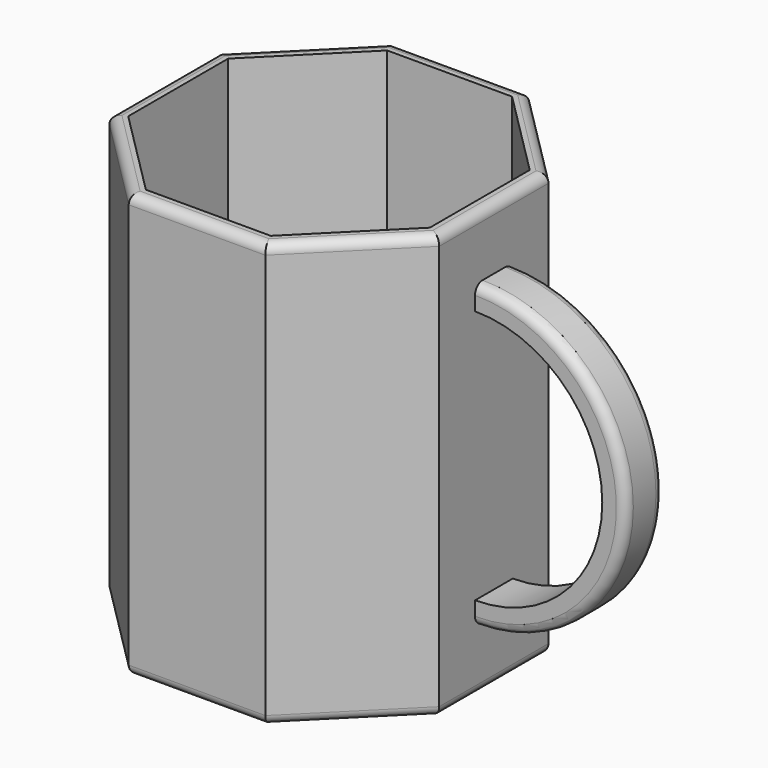
from build123d import *

# Parameters (mm, degrees)
F1_DEPTH      = 90
F2_DEPTH      = 5
F4_DEPTH      = 5
F4_DEPTH_BACK = 5
F5_R          = 2
F5_2_R        = 2


# Not quite as in the source:
# - a feature names something its author has since deleted; it is built from what else it names


with BuildPart() as f1:
    # F0 (on Top) → F1 (new body)
    with BuildSketch(Plane.XY):
        Polygon((14.4974746831, 35), (-14.4974746831, 35), (-35, 14.4974746831), (-35, -14.4974746831), (-14.4974746831, -35), (14.4974746831, -35), (35, -14.4974746831), (35, 14.4974746831), align=None)
        Polygon((-32, 13.2548339959), (-13.2548339959, 32), (13.2548339959, 32), (32, 13.2548339959), (32, -13.2548339959), (13.2548339959, -32), (-13.2548339959, -32), (-32, -13.2548339959), align=None, mode=Mode.SUBTRACT)
    extrude(amount=F1_DEPTH)

    # F5
    f5_edges = [f1.edges().sort_by_distance(p)[0] for p in [
        (24.748737, 24.748737, 90),
        (0, 35, 90),
        (-24.748737, 24.748737, 90),
        (-35, 0, 90),
        (-24.748737, -24.748737, 90),
        (0, -35, 90),
        (24.748737, -24.748737, 90),
        (35, 0, 90),
        (35, 0, 0),
        (24.748737, 24.748737, 0),
        (0, 35, 0),
        (-24.748737, 24.748737, 0),
        (-35, 0, 0),
        (-24.748737, -24.748737, 0),
        (0, -35, 0),
        (24.748737, -24.748737, 0),
    ]]
    fillet(f5_edges, radius=F5_R)


with BuildPart() as f2:
    # F0 (on Top) → F2 (new body)
    with BuildSketch(Plane.XY):
        Polygon((13.2548339959, 32), (-13.2548339959, 32), (-32, 13.2548339959), (-32, -13.2548339959), (-13.2548339959, -32), (13.2548339959, -32), (32, -13.2548339959), (32, 13.2548339959), align=None)
    extrude(amount=F2_DEPTH)


with BuildPart() as f4:
    # F3 (on Front) → F4 (new body, two sides)
    with BuildSketch(Plane.XZ) as f4_sk:
        with BuildLine():
            ThreePointArc((35, 13), (67, 45), (35, 77))
            Line((35, 77), (35, 72))
            ThreePointArc((35, 72), (62, 45), (35, 18))
            Line((35, 18), (35, 13))
        make_face()
    extrude(amount=F4_DEPTH)
    extrude(f4_sk.sketch, amount=-F4_DEPTH_BACK)

    # F5#2
    f5_2_edges = [f4.edges().sort_by_distance(p)[0] for p in [
        (67, -5, 45),
        (67, 5, 45),
    ]]
    fillet(f5_2_edges, radius=F5_2_R)


solid = Compound([f1.part, f2.part, f4.part])
